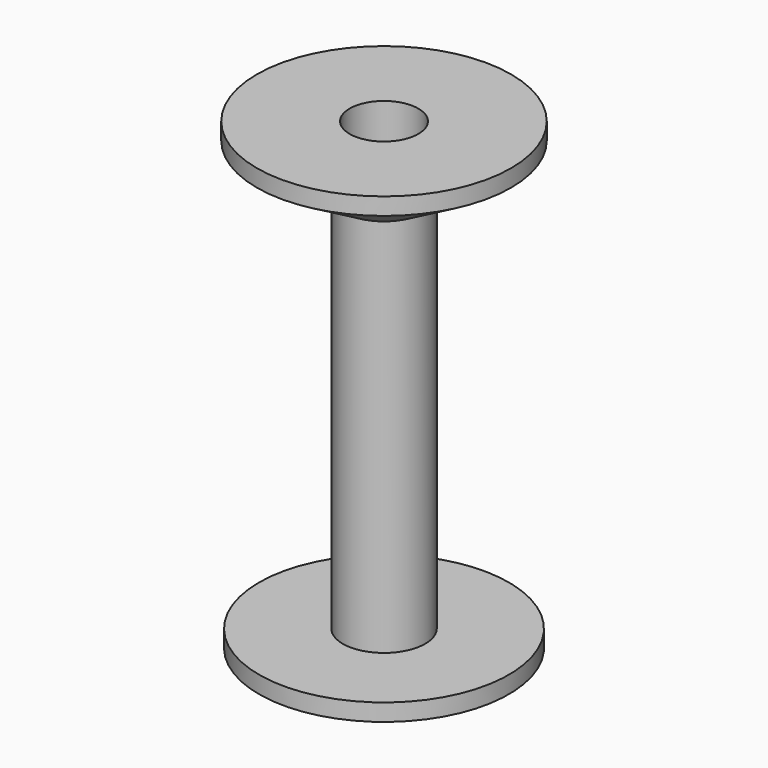
from build123d import *

# Parameters (mm, degrees)
F2_SIZE2 = 5.773493
F2_SIZE  = 9.99999


# Not quite as in the source:
# - a fillet or chamfer is up to 0.001 mm smaller than in the source, because OpenCascade refuses the exact size


with BuildPart() as f1:
    # F0 (on Front) → F1 (revolve)
    with BuildSketch(Plane.XZ):
        Polygon((-14.5480483851, 0), (-4, 0), (-4, 54), (-14.8, 54), (-14.8, 52), (-4.8, 52), (-4.8, 2), (-14.5480483851, 2), align=None)
    revolve(axis=Axis((0, 0, 27), (0, 0, -1)))

    # F2 (size 10 and 5.7735026919 in the source; OpenCascade refuses exactly that, so slightly less here)
    f2_edges = [f1.edges().sort_by_distance(p)[0] for p in [
        (4.8, 0, 52),
    ]]
    chamfer(f2_edges, length=F2_SIZE, length2=F2_SIZE2)


solid = f1.part
